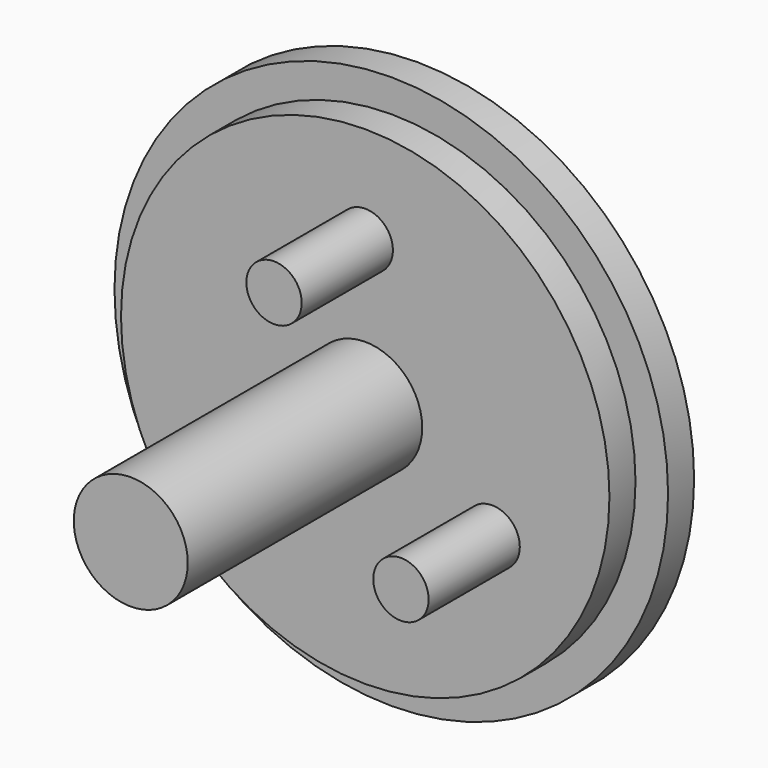
from build123d import *

# Parameters (mm, degrees)
F0_R     = 0.85
F1_DEPTH = 4.5
F0_R_2   = 7.5
F0_R_3   = 1.75
F2_DEPTH = 1
F0_R_4   = 8.5
F3_DEPTH = 1
F4_DEPTH = 10


with BuildPart() as f1:
    # F0 (on Front) → F1 (new body)
    with BuildSketch(Plane.XZ):
        with Locations((0, 4.5)):
            Circle(F0_R)
    extrude(amount=F1_DEPTH)


with BuildPart() as f1b:
    # F0 (on Front) → F1, piece 2 (new body)
    with BuildSketch(Plane.XZ):
        with Locations((-3.897114317, -2.25)):
            Circle(F0_R)
    extrude(amount=F1_DEPTH)


with BuildPart() as f1c:
    # F0 (on Front) → F1, piece 3 (new body)
    with BuildSketch(Plane.XZ):
        with Locations((3.897114317, -2.25)):
            Circle(F0_R)
    extrude(amount=F1_DEPTH)


with BuildPart() as f2:
    # F0 (on Front) → F2 (new body)
    with BuildSketch(Plane.XZ):
        Circle(F0_R_2)
        with Locations((-3.897114317, -2.25)):
            Circle(F0_R, mode=Mode.SUBTRACT)
        with Locations((3.897114317, -2.25)):
            Circle(F0_R, mode=Mode.SUBTRACT)
        Circle(F0_R_3, mode=Mode.SUBTRACT)
        with Locations((0, 4.5)):
            Circle(F0_R, mode=Mode.SUBTRACT)
    extrude(amount=F2_DEPTH)

    # F0 (on Front) → F4 (join)
    with BuildSketch(Plane.XZ):
        Circle(F0_R_3)
    extrude(amount=F4_DEPTH)


with BuildPart() as f3:
    # F0 (on Front) → F3 (new body)
    with BuildSketch(Plane.XZ):
        Circle(F0_R_4)
        Circle(F0_R_2, mode=Mode.SUBTRACT)
        Circle(F0_R_2)
        with Locations((-3.897114317, -2.25)):
            Circle(F0_R, mode=Mode.SUBTRACT)
        with Locations((3.897114317, -2.25)):
            Circle(F0_R, mode=Mode.SUBTRACT)
        Circle(F0_R_3, mode=Mode.SUBTRACT)
        with Locations((0, 4.5)):
            Circle(F0_R, mode=Mode.SUBTRACT)
        Circle(F0_R_3)
        with Locations((3.897114317, -2.25)):
            Circle(F0_R)
        with Locations((-3.897114317, -2.25)):
            Circle(F0_R)
        with Locations((0, 4.5)):
            Circle(F0_R)
    extrude(amount=-F3_DEPTH)


solid = Compound([f1.part, f1b.part, f1c.part, f2.part, f3.part])
